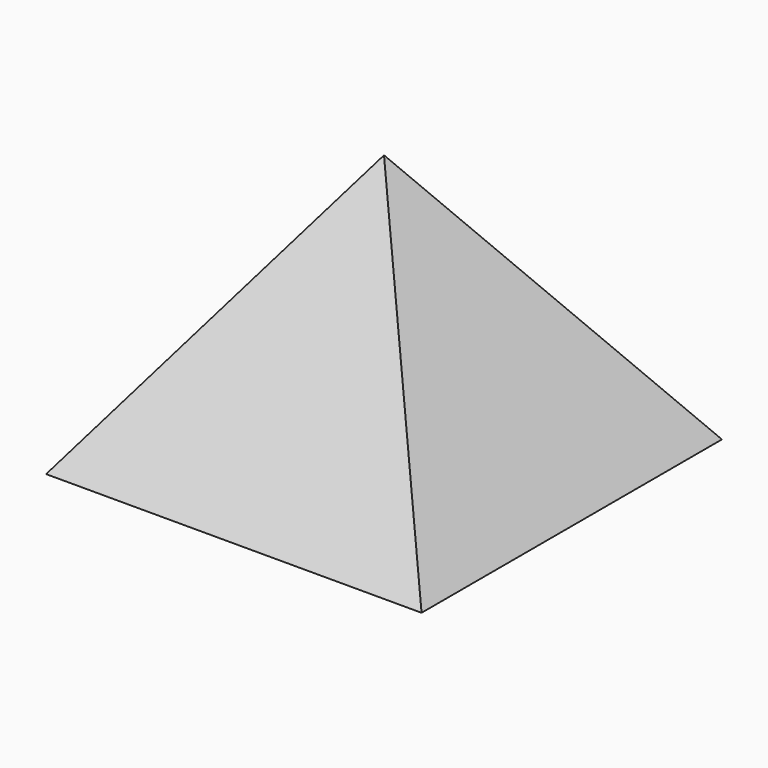
from build123d import *

# Parameters (mm, degrees)
F2_W      = 90
F2_H      = 90
F7_W      = 82
F7_H      = 82
F9_W      = 1.180001
F9_H      = 1.870001
F9_W_2    = 1.18
F9_H_2    = 4.060001
F9_W_3    = 10.110001
F9_H_3    = 1.18
F9_W_4    = 6.670001
F10_DEPTH = 2
F13_W     = 66
F13_H     = 66


# Not quite as in the source:
# - the dataset's text gives a spline's control points without its knots; the knots are read off the source's solid


with BuildPart() as f3:
    # F2 (on Top) → F3 section 0
    with BuildSketch(Plane.XY, mode=Mode.PRIVATE) as f3_s0:
        Rectangle(F2_W, F2_H)
    loft([f3_s0.sketch, Vertex(0, 0, 63.6368)])

    # F7 (on face) → F8 section 0
    with BuildSketch(Plane.XY, mode=Mode.PRIVATE) as f8_s0:
        Rectangle(F7_W, F7_H)
    loft([f8_s0.sketch, Vertex(0, 0, 58)], mode=Mode.SUBTRACT)

    # F9 (on face) → F10 (cut)
    with BuildSketch(Plane(origin=(-29.9991167733, 0, 21.2135156827), x_dir=(0, -1, 0), z_dir=(-0.8164845616, 0, 0.5773672666))):
        Polygon((21.9697801374, -21.1938021154), (23.5597841374, -21.1938021154), (28.7397811374, -15.0950853876), (28.7397811374, -19.0038021154), (29.9197811374, -19.0038021154), (29.9197811374, -14.9538011154), (28.8597821374, -14.9538011154), (28.7397811374, -14.9538011154), (22.2197811374, -14.9538011154), (21.2197821374, -16.1338011154), (26.2597841374, -16.1338011154), align=None)
        with Locations((31.4797826374, -18.0688016154)):
            Rectangle(F9_W, F9_H)
        with Locations((33.6297791374, -19.1638016154)):
            Rectangle(F9_W_2, F9_H_2)
        Polygon((12.0897811374, -21.1938021154), (20.2597801374, -21.1938021154), (20.8297821374, -20.0438011154), (18.3297821374, -14.9538011154), (13.9597791374, -14.9538011154), (11.4997811374, -19.9838021154), align=None)
        Polygon((19.3697831374, -20.0138021154), (12.9197831374, -20.0138021154), (14.8197791374, -16.1338011154), (17.4797821374, -16.1338011154), align=None, mode=Mode.SUBTRACT)
        with BuildLine():
            Line((5.2997801374, -14.9538011154), (5.2997801374, -16.6038011154))
            add(Edge.make_bspline(
                [(4.1407171374, -16.7288011154), (4.3252931374, -16.7141861154), (4.7128221374, -16.6835011154), (5.0980381374, -16.6311951154), (5.2997801374, -16.6038011154)],
                knots=[0, 0, 0, 0, 0.555346, 1.165986, 1.165986, 1.165986, 1.165986], degree=3))
            add(Edge.make_bspline(
                [(3.2325931374, -16.7738011154), (3.3718421374, -16.7690131154), (3.6747741374, -16.7585981154), (3.9772701374, -16.7392531154), (4.1407171374, -16.7288011154)],
                knots=[0, 0, 0, 0, 0.417971, 0.909282, 0.909282, 0.909282, 0.909282], degree=3))
            add(Edge.make_bspline(
                [(2.4297801374, -16.7638011154), (2.5552081374, -16.7691171154), (2.8227031374, -16.7804551154), (3.0904121374, -16.7761091154), (3.2325931374, -16.7738011154)],
                knots=[0, 0, 0, 0, 0.376537, 0.803027, 0.803027, 0.803027, 0.803027], degree=3))
            Line((2.4297801374, -16.7638011154), (1.2497801374, -16.7638011154))
            Line((1.2497801374, -16.7638011154), (1.2497801374, -21.1938021154))
            Line((1.2497801374, -21.1938021154), (10.6597801374, -21.1938021154))
            Line((10.6597801374, -21.1938021154), (10.6597801374, -20.0138021154))
            Line((10.6597801374, -20.0138021154), (6.4797801374, -20.0138021154))
            Line((6.4797801374, -20.0138021154), (6.4797801374, -17.6491141154))
            add(Edge.make_bspline(
                [(8.6047791374, -17.0530201154), (8.2523501374, -17.1763541154), (7.5565571374, -17.4198491154), (6.8355751374, -17.5733591154), (6.4797801374, -17.6491141154)],
                knots=[0, 0, 0, 0, 1.118887, 2.208999, 2.208999, 2.208999, 2.208999], degree=3))
            add(Edge.make_bspline(
                [(10.6597801374, -16.1361451154), (10.3259741374, -16.3048751154), (9.6557671374, -16.6436461154), (8.9560111374, -16.9162101154), (8.6047791374, -17.0530201154)],
                knots=[0, 0, 0, 0, 1.121359, 2.251432, 2.251432, 2.251432, 2.251432], degree=3))
            Line((10.6597801374, -16.1361451154), (10.6597801374, -14.9538011154))
            add(Edge.make_bspline(
                [(8.5247801374, -15.8638011154), (8.8834781374, -15.7390181154), (9.6157961374, -15.4842611154), (10.3070901374, -15.1330071154), (10.6597801374, -14.9538011154)],
                knots=[0, 0, 0, 0, 1.137935, 2.323212, 2.323212, 2.323212, 2.323212], degree=3))
            add(Edge.make_bspline(
                [(6.4797801374, -16.4038011154), (6.8146711374, -16.3298001154), (7.5036441374, -16.1775551154), (8.1781381374, -15.9703101154), (8.5247801374, -15.8638011154)],
                knots=[0, 0, 0, 0, 1.028459, 2.115858, 2.115858, 2.115858, 2.115858], degree=3))
            Line((6.4797801374, -16.4038011154), (6.4797801374, -14.9538011154))
            Line((6.4797801374, -14.9538011154), (5.2997801374, -14.9538011154))
        make_face()
        with BuildLine():
            Line((5.2997801374, -20.0138021154), (2.4297801374, -20.0138021154))
            Line((2.4297801374, -20.0138021154), (2.4297801374, -17.9538021154))
            add(Edge.make_bspline(
                [(3.2525921374, -17.9638011154), (3.1087451374, -17.9660571154), (2.8343741374, -17.9703591154), (2.5602071374, -17.9591391154), (2.4297801374, -17.9538021154)],
                knots=[0, 0, 0, 0, 0.431492, 0.823018, 0.823018, 0.823018, 0.823018], degree=3))
            add(Edge.make_bspline(
                [(4.1557951374, -17.9288011154), (3.9935791374, -17.9363501154), (3.6926011374, -17.9503551154), (3.3914391374, -17.9595581154), (3.2525921374, -17.9638011154)],
                knots=[0, 0, 0, 0, 0.487164, 0.903894, 0.903894, 0.903894, 0.903894], degree=3))
            add(Edge.make_bspline(
                [(5.2997801374, -17.8238011154), (5.1009381374, -17.8479581154), (4.7206281374, -17.8941601154), (4.3382501374, -17.9176111154), (4.1557951374, -17.9288011154)],
                knots=[0, 0, 0, 0, 0.600755, 1.14902, 1.14902, 1.14902, 1.14902], degree=3))
            Line((5.2997801374, -17.8238011154), (5.2997801374, -20.0138021154))
        make_face(mode=Mode.SUBTRACT)
        Polygon((-7.2802218626, -14.9538011154), (-9.6202208626, -19.7238021154), (-11.9602208626, -14.9538011154), (-13.3902208626, -14.9538011154), (-10.3302198626, -21.1938021154), (-8.9002208626, -21.1938021154), (-6.4202218626, -16.1338011154), (-5.8402208626, -16.1338011154), (-5.8402208626, -21.1938021154), (-4.6602208626, -21.1938021154), (-4.6602208626, -16.1338011154), (-3.9402198626, -16.1338011154), (-3.9402198626, -14.9538011154), align=None)
        with Locations((-18.7952213626, -15.5438011154)):
            Rectangle(F9_W_3, F9_H_3)
        with Locations((-18.7952213626, -18.0738011154)):
            Rectangle(F9_W_4, F9_H_3)
        with Locations((-18.7952213626, -20.6038021154)):
            Rectangle(F9_W_3, F9_H_3)
        Polygon((-33.1302218626, -18.0738021154), (-30.4802218626, -21.1938021154), (-27.3102218626, -21.1938021154), (-24.6602208626, -18.0738021154), (-26.2502218626, -18.0738021154), (-28.3002218626, -20.4938021154), (-28.3002218626, -14.9538011154), (-29.4802218626, -14.9538011154), (-29.4802218626, -20.4938021154), (-31.5402218626, -18.0738021154), align=None)
    extrude(amount=-F10_DEPTH, mode=Mode.SUBTRACT)

    # F13 (on offset) → F14 section 0
    with BuildSketch(Plane.XY.offset(12), mode=Mode.PRIVATE) as f14_s0:
        Rectangle(F13_W, F13_H)
    loft([Vertex(0, 0, 58), f14_s0.sketch])

    # F11 (on offset) → F15 (revolve, cut)
    with BuildSketch(Plane.XY.offset(25)):
        with BuildLine():
            Line((0, -20), (0, 20))
            ThreePointArc((0, 20), (-20, 0), (0, -20))
        make_face()
    revolve(axis=Axis((0, 0, 25), (0, 1, 0)), mode=Mode.SUBTRACT)


solid = f3.part
